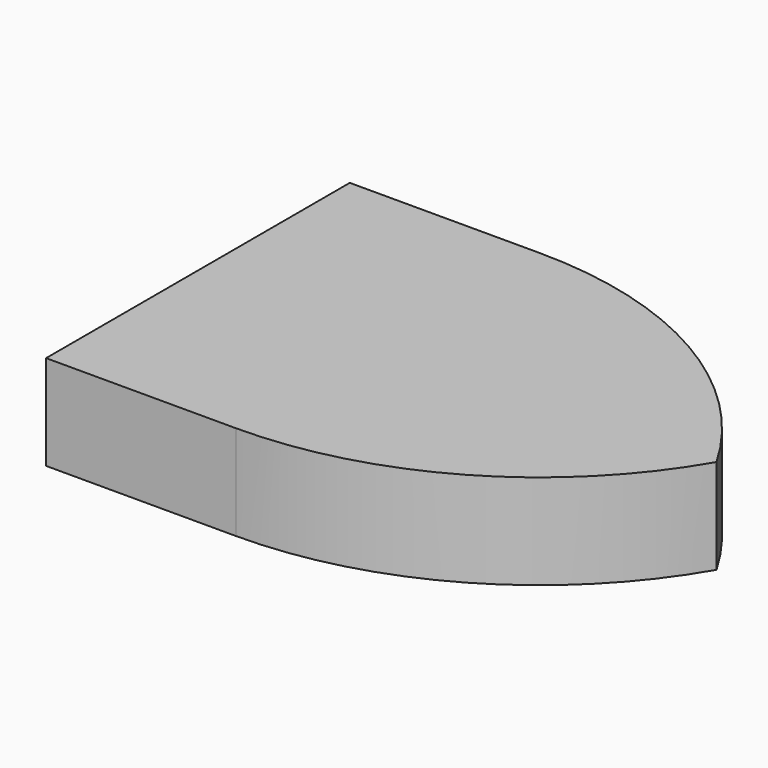
from build123d import *

# Parameters (mm, degrees)
F0_W        = 60
F0_H        = 10
F1_DEPTH    = 40
F2_T1_DEPTH = 210


# Not quite as in the source:
# - a fillet or chamfer that OpenCascade refuses, or shapes differently, is made with other operations: its cross-section is extruded or revolved along the edge and cut away or added


with BuildPart() as f1:
    # F0 (on Front) → F1 (new body)
    with BuildSketch(Plane.XZ):
        with Locations((2.7074571699, -10.2079533711)):
            Rectangle(F0_W, F0_H)
    extrude(amount=F1_DEPTH)

    # F2: fillet of radius 40 on 2 edges, made by hand

    # F2_s2 → F2_t1 (cut)
    with BuildSketch(Plane.XY.offset(-115.2079533711)):
        with BuildLine():
            ThreePointArc((32.7074571699, 0), (20.9917284174, -28.2842712475), (-7.2925428301, -40))
            Line((-7.2925428301, -40), (32.7074571699, -40))
            Line((32.7074571699, -40), (32.7074571699, 0))
        make_face()
        with BuildLine():
            ThreePointArc((32.7074571699, -40), (20.9917284174, -11.7157287525), (-7.2925428301, 0))
            Line((-7.2925428301, 0), (32.7074571699, 0))
            Line((32.7074571699, 0), (32.7074571699, -40))
        make_face()
    extrude(amount=F2_T1_DEPTH, mode=Mode.SUBTRACT)


solid = f1.part
